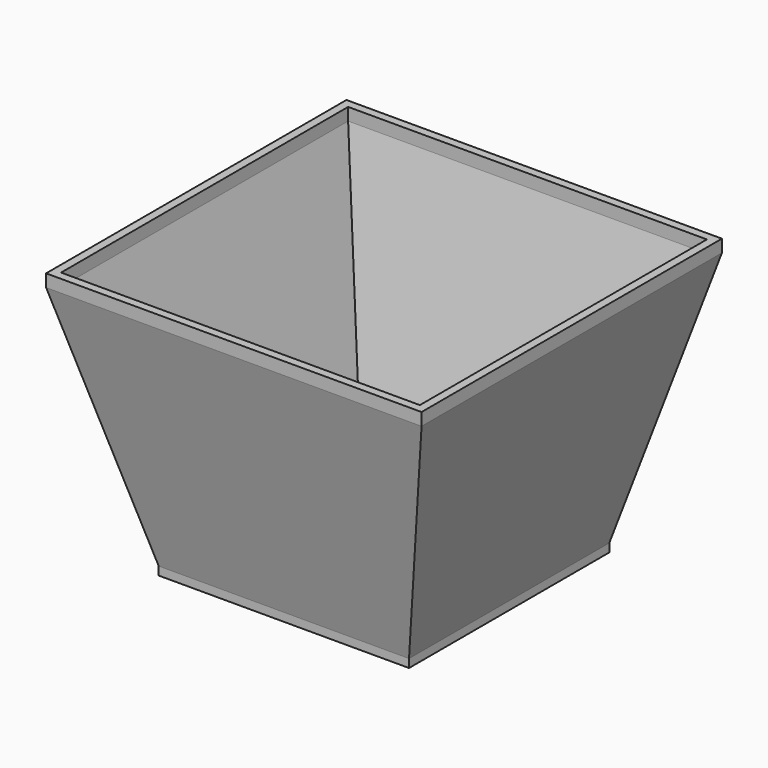
from build123d import *

# Parameters (mm, degrees)
F0_W     = 28
F0_H     = 28
F7_DEPTH = 1
F8_DEPTH = 1.5


with BuildPart() as f3:
    # F2 (on offset) → F3 section 0
    with BuildSketch(Plane.XY.offset(30)):
        Polygon((22.5, -22.5), (21.5, -21.5), (-21.5, -21.5), (-22.5, -22.5), align=None)
    # F0 (on Top) → F3 section 1
    with BuildSketch(Plane.XY):
        Polygon((15, -15), (14, -14), (-14, -14), (-15, -15), align=None)
    loft()

    # F0 (on Top) → F4 section 0
    with BuildSketch(Plane.XY):
        Polygon((14, 14), (14, -14), (15, -15), (15, 15), align=None)
    # F2 (on offset) → F4 section 1
    with BuildSketch(Plane.XY.offset(30)):
        Polygon((21.5, 21.5), (21.5, -21.5), (22.5, -22.5), (22.5, 22.5), align=None)
    loft()

    # F0 (on Top) → F5 section 0
    with BuildSketch(Plane.XY):
        Polygon((-14, 14), (14, 14), (15, 15), (-15, 15), align=None)
    # F2 (on offset) → F5 section 1
    with BuildSketch(Plane.XY.offset(30)):
        Polygon((-21.5, 21.5), (21.5, 21.5), (22.5, 22.5), (-22.5, 22.5), align=None)
    loft()

    # F0 (on Top) → F6 section 0
    with BuildSketch(Plane.XY):
        Polygon((-15, -15), (-14, -14), (-14, 14), (-15, 15), align=None)
    # F2 (on offset) → F6 section 1
    with BuildSketch(Plane.XY.offset(30)):
        Polygon((-22.5, -22.5), (-21.5, -21.5), (-21.5, 21.5), (-22.5, 22.5), align=None)
    loft()

    # F0 (on Top) → F7 (join)
    with BuildSketch(Plane.XY):
        Polygon((-14, 14), (14, 14), (15, 15), (-15, 15), align=None)
        Polygon((-15, -15), (-14, -14), (-14, 14), (-15, 15), align=None)
        Polygon((15, -15), (14, -14), (-14, -14), (-15, -15), align=None)
        Polygon((14, 14), (14, -14), (15, -15), (15, 15), align=None)
        Rectangle(F0_W, F0_H)
    extrude(amount=-F7_DEPTH)

    # F2 (on offset) → F8 (join)
    with BuildSketch(Plane.XY.offset(30)):
        Polygon((22.5, -22.5), (21.5, -21.5), (-21.5, -21.5), (-22.5, -22.5), align=None)
        Polygon((21.5, 21.5), (21.5, -21.5), (22.5, -22.5), (22.5, 22.5), align=None)
        Polygon((-21.5, 21.5), (21.5, 21.5), (22.5, 22.5), (-22.5, 22.5), align=None)
        Polygon((-22.5, -22.5), (-21.5, -21.5), (-21.5, 21.5), (-22.5, 22.5), align=None)
    extrude(amount=F8_DEPTH)


solid = f3.part
